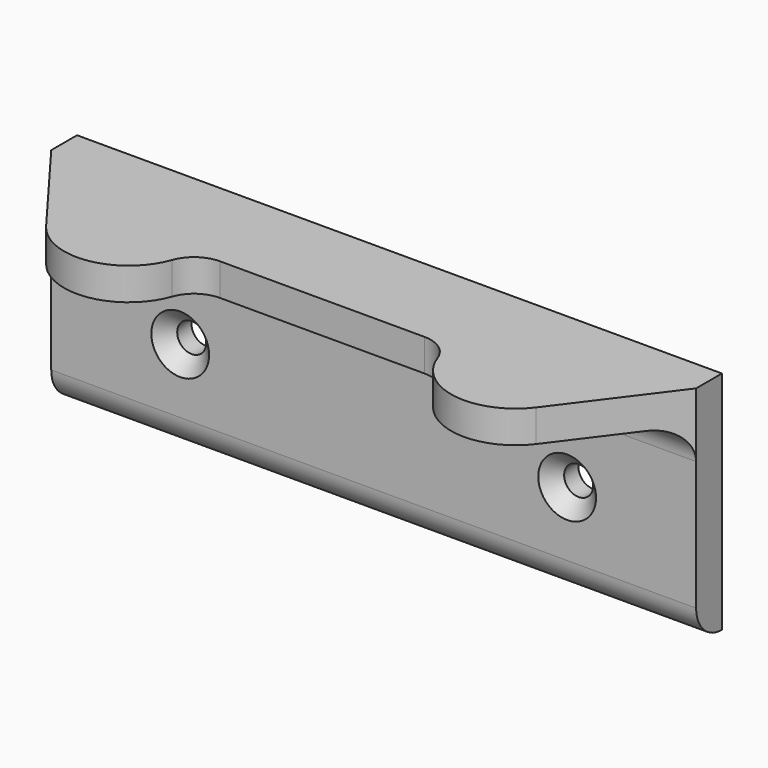
from build123d import *

# Parameters (mm, degrees)
F0_W           = 100
F0_H           = 35
F1_DEPTH       = 5
F3_DEPTH       = 5
F4_R           = 5
F5_R           = 4.99999
F7_D           = 4.5
F7_CSINK_D     = 8.96
F7_CSINK_ANGLE = 90


# Not quite as in the source:
# - a fillet or chamfer is up to 0.001 mm smaller than in the source, because OpenCascade refuses the exact size


with BuildPart() as f1:
    # F0 (on Front) → F1 (new body)
    with BuildSketch(Plane.XZ):
        with Locations((0, 7.5)):
            Rectangle(F0_W, F0_H)
    extrude(amount=F1_DEPTH)

    # F2 (on face) → F3 (join)
    with BuildSketch(Plane.XY.offset(25)):
        with BuildLine():
            Line((-50, -5), (-38, -21))
            ThreePointArc((-38, -21), (-26.8377223398, -24.4868329805), (-20, -15))
            Line((-20, -15), (20, -15))
            ThreePointArc((20, -15), (26.8377223398, -24.4868329805), (38, -21))
            Line((38, -21), (50, -5))
            Line((50, -5), (-50, -5))
        make_face()
    extrude(amount=-F3_DEPTH)

    # F4
    f4_edges = [f1.edges().sort_by_distance(p)[0] for p in [
        (-20, -15, 22.5),
        (0, -5, 20),
        (20, -15, 22.5),
    ]]
    fillet(f4_edges, radius=F4_R)

    # F5 (radius 5 in the source; OpenCascade refuses exactly that, so slightly less here)
    f5_edges = [f1.edges().sort_by_distance(p)[0] for p in [
        (0, -5, -10),
    ]]
    fillet(f5_edges, radius=F5_R)

    # F7 (through all)
    with Locations(Plane.XZ.offset(5)):
        with Locations((-30, 5), (30, 5)):
            CounterSinkHole(F7_D / 2, F7_CSINK_D / 2, counter_sink_angle=F7_CSINK_ANGLE)


solid = f1.part
